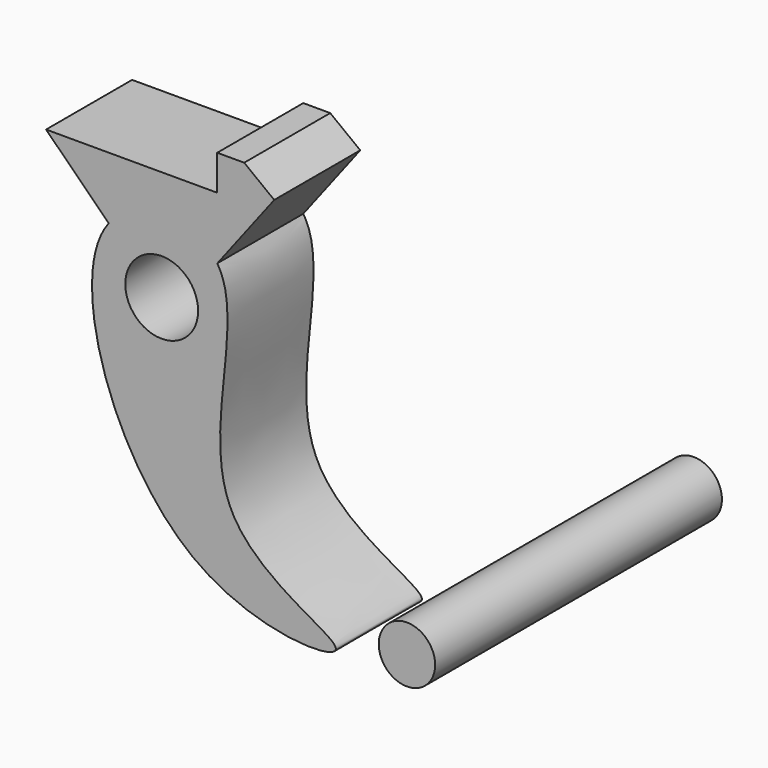
from build123d import *

# Parameters (mm, degrees)
F0_R     = 2.5801610902
F1_DEPTH = 7.62
F0_R_2   = 1.9983681338
F2_DEPTH = 17.78


with BuildPart() as f1:
    # F0 (on Front) → F1 (new body)
    with BuildSketch(Plane.XZ):
        with BuildLine():
            add(Edge.make_bspline(
                [(-26.3524726033, 38.1400510669), (-27.8596560993, 40.4321397588), (-32.1477926679, 40.574573371), (-34.0432301164, 38.1376333535)],
                knots=[0.8409342104, 0.8409342104, 0.8409342104, 0.8409342104, 1, 1, 1, 1], degree=3))
            add(Edge.make_bspline(
                [(-34.0432301164, 38.1376333535), (-37.0936300965, 34.2157725783), (-31.6862921183, 15.9960381182), (-12.3480035084, 15.9505507078), (-30.3028477282, 21.5025635075), (-24.2301882963, 34.912531741), (-26.3524726033, 38.1400510669)],
                knots=[0, 0, 0, 0, 0.255990659, 0.4399097759, 0.6169516429, 0.8409342104, 0.8409342104, 0.8409342104, 0.8409342104], degree=3))
        make_face()
        with Locations((-30.2872788161, 34.7385704517)):
            Circle(F0_R, mode=Mode.SUBTRACT)
        with BuildLine():
            Line((-38.4799912572, 42.5488176732), (-34.0432301164, 38.1376333535))
            add(Edge.make_bspline(
                [(-26.3524726033, 38.1400510669), (-27.8596560993, 40.4321397588), (-32.1477926679, 40.574573371), (-34.0432301164, 38.1376333535)],
                knots=[0.8409342104, 0.8409342104, 0.8409342104, 0.8409342104, 1, 1, 1, 1], degree=3))
            Line((-26.3524726033, 38.1400510669), (-22.3134607077, 43.4132032096))
            Line((-22.3134607077, 43.4132032096), (-24.4417442845, 45.043378568))
            Line((-24.4417442845, 45.043378568), (-26.3524726033, 42.5488176732))
            Line((-26.3524726033, 42.5488176732), (-38.4799912572, 42.5488176732))
        make_face()
        Polygon((-26.3524726033, 45.043378568), (-26.3524726033, 42.5488176732), (-24.4417442845, 45.043378568), align=None)
    extrude(amount=F1_DEPTH)


with BuildPart() as f1b:
    # F0 (on Front) → F1, piece 2 (new body)
    with BuildSketch(Plane.XZ):
        with Locations((1.3145125704, 29.9708880484)):
            Circle(F0_R_2)
    extrude(amount=F1_DEPTH)

    # F2 (add): a face of the model
    f2_faces = [f1b.faces().sort_by_distance(p)[0] for p in [
        (1.3145125704, -7.62, 29.9708880484),
    ]]
    extrude(f2_faces, amount=F2_DEPTH)


solid = Compound([f1.part, f1b.part])
